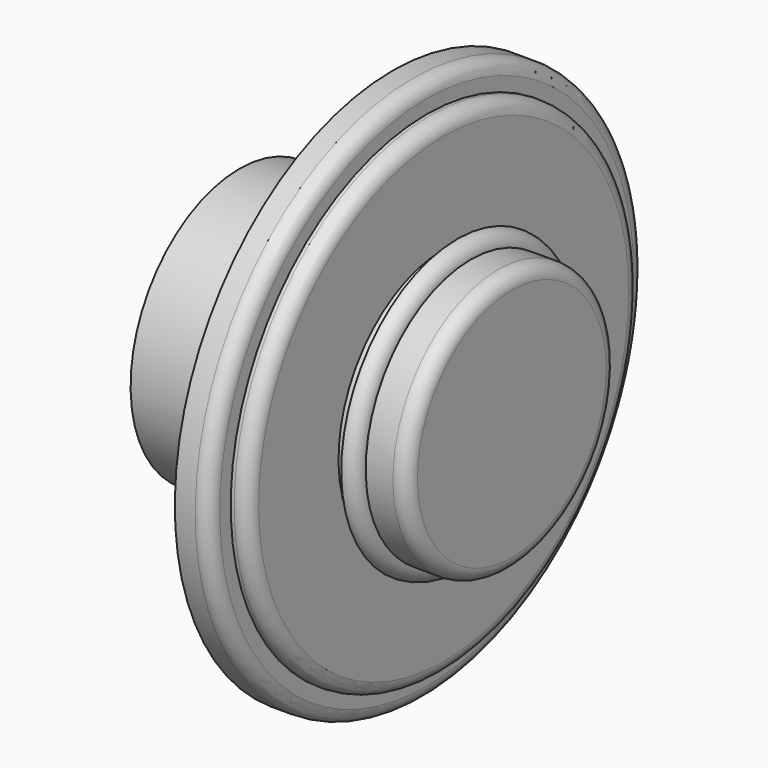
from build123d import *

# Parameters (mm, degrees)
F2_R = 0.99999


# Not quite as in the source:
# - a fillet or chamfer is up to 0.001 mm smaller than in the source, because OpenCascade refuses the exact size


with BuildPart() as f1:
    # F0 (on Front) → F1 (revolve)
    with BuildSketch(Plane.XZ):
        Polygon((0, 10), (0, 0), (20, 0), (20, 9.6603445709), (17, 9.6603445709), (17, 10.6603445709), (16, 10.6603445709), (16, 9.6603445709), (15, 9.6603445709), (15, 17.993060872), (13.75, 17.993060872), (13.75, 20), (11.25, 20), (11.25, 18), (10, 18), (10, 10), align=None)
    revolve(axis=Axis((10, 0, 0), (-1, 0, 0)))

    # F2 (radius 1 in the source; OpenCascade refuses exactly that, so slightly less here)
    f2_edges = [f1.edges().sort_by_distance(p)[0] for p in [
        (20, 0, -9.660345),
        (17, 0, -10.660345),
        (15, 0, -17.993061),
        (13.75, 0, -20),
    ]]
    fillet(f2_edges, radius=F2_R)


solid = f1.part
